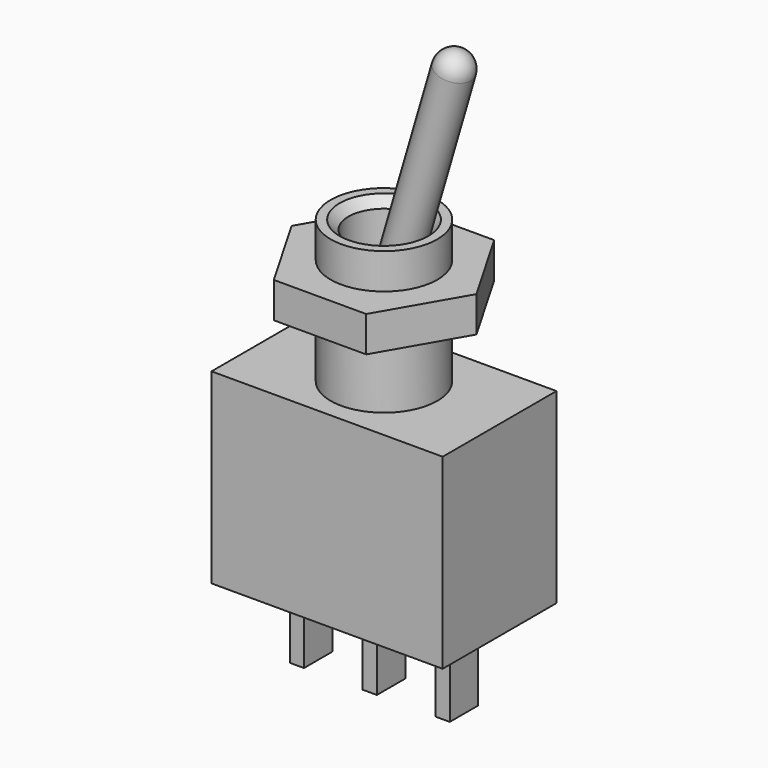
from build123d import *

# Parameters (mm, degrees)
F1_DEPTH    = 4
F2_W        = 3
F2_H        = 4.5
F3_DEPTH    = 13.001
F4_R        = 3
F5_DEPTH    = 8
F8_DEPTH    = 2
F9_T        = 1
F9_T3_DEPTH = 2.8
F9_T5_DEPTH = 4
F9_T7_DEPTH = 2.8
F9_T9_DEPTH = 2.8
F11_SIZE    = 0.5
F13_R       = 1
F14_DEPTH   = 15
F15_R       = 1


# Not quite as in the source:
# - a shell that OpenCascade refuses in one call is made with other operations: the cavity is built on its own and cut out


with BuildPart() as f1:
    # F0 (on Front) → F1 (new body, symmetric)
    with BuildSketch(Plane.XZ):
        Polygon((6.5, -13.8051480774), (6.5, -3.3051480774), (-6.5, -3.3051480774), (-6.5, -13.8051480774), (-4.5, -13.8051480774), (-4.5, -18.3051480774), (-3.7, -18.3051480774), (-3.7, -13.8051480774), (-0.4, -13.8051480774), (-0.4, -18.3051480774), (0.4, -18.3051480774), (0.4, -13.8051480774), (3.7, -13.8051480774), (3.7, -18.3051480774), (4.5, -18.3051480774), (4.5, -13.8051480774), align=None)
    extrude(amount=F1_DEPTH, both=True)

    # F2 (on face) → F3 (cut, through all)
    with BuildSketch(Plane.YZ.offset(6.5)):
        with Locations((-2.5, -16.0551480774)):
            Rectangle(F2_W, F2_H)
        with Locations((2.5, -16.0551480774)):
            Rectangle(F2_W, F2_H)
    extrude(amount=-F3_DEPTH, mode=Mode.SUBTRACT)

    # F4 (on face) → F5 (join)
    with BuildSketch(Plane.XY.offset(-3.3051480774)):
        Circle(F4_R)
    extrude(amount=F5_DEPTH)

    # F7 (on offset) → F8 (join)
    with BuildSketch(Plane.XY.offset(0.6948519226)):
        Polygon((2.5980762114, -4.5), (5.1961524227, 0), (2.5980762114, 4.5), (-2.5980762114, 4.5), (-5.1961524227, 0), (-2.5980762114, -4.5), align=None)
    extrude(amount=F8_DEPTH)

    # F9: shell of thickness 1, made by hand


with BuildPart() as f9_core1:
    # F9_t2: copy of F1
    add(f1.part)

    # the walls: a layer under each face that stays
    f9_faces = [f9_core1.faces().sort_by_distance(p)[0] for p in [
        (-4.3333333333, 2.6666666667, -13.8051480774),
        (6.5, 0, -8.5551480774),
        (0, -4, -8.5551480774),
        (-6.5, 0, -8.5551480774),
        (0, 4, -8.5551480774),
        (0, 1, -16.0551480774),
        (-0.4, 0, -16.0551480774),
        (0, -1, -16.0551480774),
        (0.4, 0, -16.0551480774),
        (3.7, 0, -16.0551480774),
        (4.1, -1, -16.0551480774),
        (4.5, 0, -16.0551480774),
        (4.1, 1, -16.0551480774),
        (-4.1, 1, -16.0551480774),
        (-4.5, 0, -16.0551480774),
        (-4.1, -1, -16.0551480774),
        (-3.7, 0, -16.0551480774),
        (4.3333333333, 2.6666666667, -3.3051480774),
        (0, 0, -18.3051480774),
        (4.1, 0, -18.3051480774),
        (-4.1, 0, -18.3051480774),
        (-3, 0, -1.3051480774),
        (-3.4641016151, 0, 0.6948519226),
        (-3.897114317, -2.25, 1.6948519226),
        (-3.897114317, 2.25, 1.6948519226),
        (0, -4.5, 1.6948519226),
        (0, 4.5, 1.6948519226),
        (3.897114317, -2.25, 1.6948519226),
        (3.897114317, 2.25, 1.6948519226),
        (-3.4641016151, 0, 2.6948519226),
        (-3, 0, 3.6948519226),
    ]]
    thicken(f9_faces, amount=-F9_T, mode=Mode.SUBTRACT)

    # F9_s4 → F9_t3 (cut)
    with BuildSketch(Plane.YZ.offset(-1.4)):
        Polygon((1.01, -13.8151480774), (1, -12.8051480774), (0, -12.8051480774), (0, -13.8051480774), align=None)
        Polygon((-1.01, -13.8151480774), (-1, -12.8051480774), (0, -12.8051480774), (0, -13.8051480774), align=None)
    extrude(amount=F9_T3_DEPTH, mode=Mode.SUBTRACT)

    # F9_s6 → F9_t5 (cut)
    with BuildSketch(Plane.XZ.offset(-2)):
        Polygon((-0.41, -13.8151480774), (-0.4, -12.8051480774), (0.6, -12.8051480774), (0.6, -13.8051480774), align=None)
        Polygon((0.41, -13.8151480774), (0.4, -12.8051480774), (-0.6, -12.8051480774), (-0.6, -13.8051480774), align=None)
        Polygon((3.69, -13.8151480774), (3.7, -12.8051480774), (4.7, -12.8051480774), (4.7, -13.8051480774), align=None)
        Polygon((4.51, -13.8151480774), (4.5, -12.8051480774), (3.5, -12.8051480774), (3.5, -13.8051480774), align=None)
        Polygon((-4.51, -13.8151480774), (-4.5, -12.8051480774), (-3.5, -12.8051480774), (-3.5, -13.8051480774), align=None)
        Polygon((-3.69, -13.8151480774), (-3.7, -12.8051480774), (-4.7, -12.8051480774), (-4.7, -13.8051480774), align=None)
    extrude(amount=F9_T5_DEPTH, mode=Mode.SUBTRACT)

    # F9_s8 → F9_t7 (cut)
    with BuildSketch(Plane.YZ.offset(2.7)):
        Polygon((-1.01, -13.8151480774), (-1, -12.8051480774), (0, -12.8051480774), (0, -13.8051480774), align=None)
        Polygon((1.01, -13.8151480774), (1, -12.8051480774), (0, -12.8051480774), (0, -13.8051480774), align=None)
    extrude(amount=F9_T7_DEPTH, mode=Mode.SUBTRACT)

    # F9_s10 → F9_t9 (cut)
    with BuildSketch(Plane.YZ.offset(-5.5)):
        Polygon((1.01, -13.8151480774), (1, -12.8051480774), (0, -12.8051480774), (0, -13.8051480774), align=None)
        Polygon((-1.01, -13.8151480774), (-1, -12.8051480774), (0, -12.8051480774), (0, -13.8051480774), align=None)
    extrude(amount=F9_T9_DEPTH, mode=Mode.SUBTRACT)

    # F9_s11 → F9_t12 (revolve, cut)
    with BuildSketch(Plane.XZ):
        Polygon((3.01, -3.2951480774), (3, -4.3051480774), (2, -4.3051480774), (2, -3.3051480774), align=None)
    revolve(axis=Axis((0, 0, -3.3051480774), (0, 0, 1)), mode=Mode.SUBTRACT)

    # F9_s13 → F9_t14 (revolve, cut)
    with BuildSketch(Plane.XZ):
        Polygon((3.01, 0.6848519226), (2, 0.6948519226), (2, 1.6948519226), (3, 1.6948519226), align=None)
    revolve(axis=Axis((0, 0, 0.6948519226), (0, 0, -1)), mode=Mode.SUBTRACT)

    # F9_s15 → F9_t16 (revolve, cut)
    with BuildSketch(Plane.XZ):
        Polygon((3.01, 2.7048519226), (3, 1.6948519226), (2, 1.6948519226), (2, 2.6948519226), align=None)
    revolve(axis=Axis((0, 0, 2.6948519226), (0, 0, -1)), mode=Mode.SUBTRACT)


with BuildPart() as f1_1:
    add(f1.part)

    # what is left inside the walls is the cavity
    f9_cavity = [f9_core1.part.solids().sort_by_distance(p)[0] for p in [
        (0, 2.99, -9.971815),
    ]]
    add(f9_cavity, mode=Mode.SUBTRACT)

    # F11
    f11_edges = [f1_1.edges().sort_by_distance(p)[0] for p in [
        (-2, 0, 4.694852),
    ]]
    chamfer(f11_edges, length=F11_SIZE)

    # F13 (on line) → F14 (join)
    with BuildSketch(Plane(origin=(0, 0, 0), x_dir=(0.9597844806, 0, -0.2807378684), z_dir=(0.2807378684, 0, 0.9597844806))):
        Circle(F13_R)
    extrude(amount=F14_DEPTH)

    # F15
    f15_edges = [f1_1.edges().sort_by_distance(p)[0] for p in [
        (3.251284, 0, 14.677505),
    ]]
    fillet(f15_edges, radius=F15_R)


solid = f1_1.part
